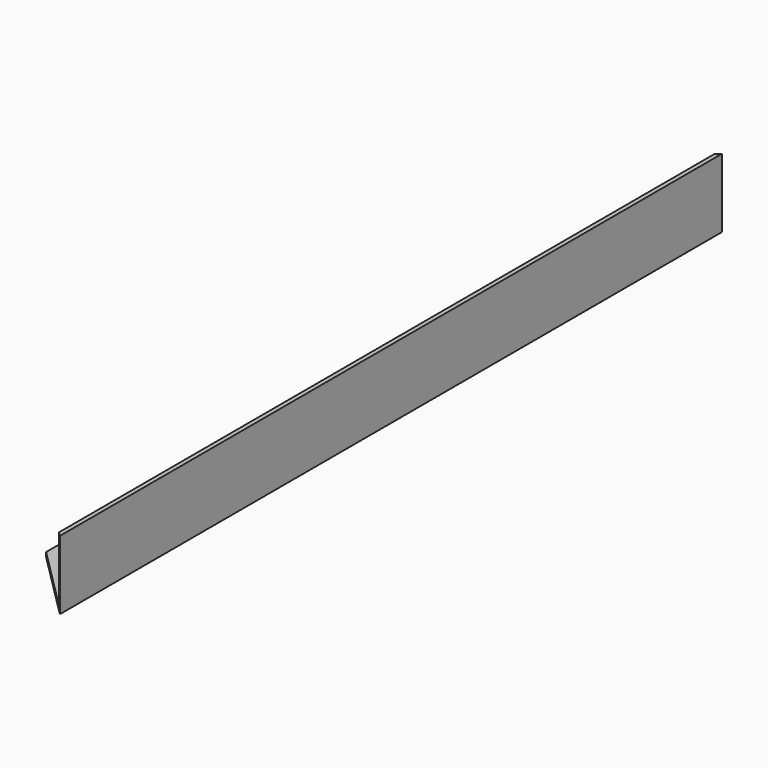
from build123d import *

# Parameters (mm, degrees)
F1_DEPTH = 304.8
F2_SIZE  = 50.79999
F3_SIZE  = 50.79999


# Not quite as in the source:
# - a fillet or chamfer is up to 0.001 mm smaller than in the source, because OpenCascade refuses the exact size


with BuildPart() as f1:
    # F0 (on Front) → F1 (new body, symmetric)
    with BuildSketch(Plane.XZ):
        Polygon((76.2, 3.175), (76.2, 0), (127, 0), (127, 50.8), (123.825, 50.8), (123.825, 3.175), align=None)
    extrude(amount=F1_DEPTH, both=True)

    # F2 (size 50.8 in the source; OpenCascade refuses exactly that, so slightly less here)
    f2_edges = [f1.edges().sort_by_distance(p)[0] for p in [
        (76.2, -304.8, 1.5875),
    ]]
    chamfer(f2_edges, length=F2_SIZE)

    # F3 (size 50.8 in the source; OpenCascade refuses exactly that, so slightly less here)
    f3_edges = [f1.edges().sort_by_distance(p)[0] for p in [
        (76.2, 304.8, 1.5875),
    ]]
    chamfer(f3_edges, length=F3_SIZE)


solid = f1.part
